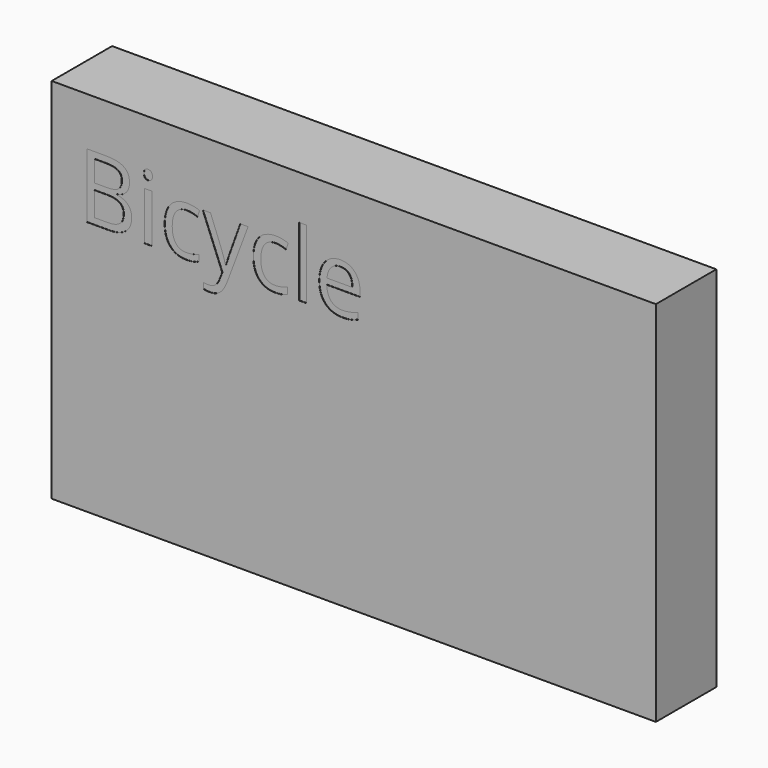
from build123d import *

# Parameters (mm, degrees)
F0_W         = 1840
F0_H         = 1120
F1_DEPTH     = 230
F2_TEXT_SIZE = 275.4043373797
F3_DEPTH     = 1


# Not quite as in the source:
# - Text() gives the source's letters only with a copy of the font that has no kerning and outlines rounded to 1/6400 em; it was checked with that copy


with BuildPart() as f1:
    # F0 (on Front) → F1 (new body)
    with BuildSketch(Plane.XZ):
        with Locations((920, 560)):
            Rectangle(F0_W, F0_H)
    extrude(amount=F1_DEPTH)

    # F2 (on face) → F3 (cut)
    with BuildSketch(Plane.XZ.offset(230)):
        with Locations((80.3709104657, 776.4132618904)):
            Text('Bicycle', F2_TEXT_SIZE, font='Open Sans', text_align=(TextAlign.LEFT, TextAlign.BOTTOM))
    extrude(amount=-F3_DEPTH, mode=Mode.SUBTRACT)


solid = f1.part
